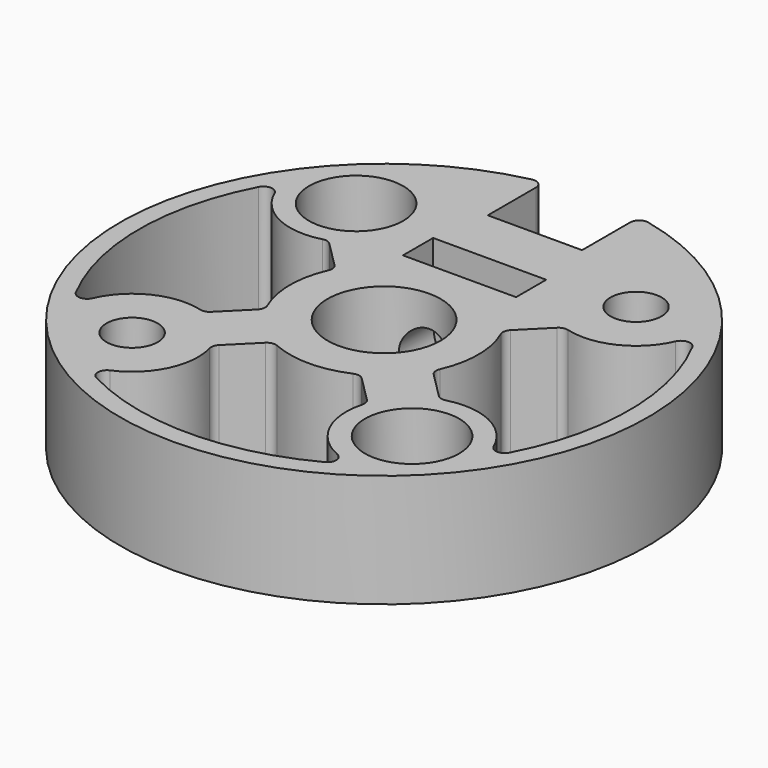
from build123d import *

# Parameters (mm, degrees)
F0_R            = 2.15265
F0_R_2          = 4.7625
F0_W            = 9.525
F0_H            = 3.175
F1_DEPTH        = 9.525
F2_R            = 2.15265
F3_REACH        = 44.1896136501
F6_R            = 3.96875
F7_DEPTH        = 6.35
F9_DEPTH        = 9.525
F9_COPIES_COUNT = 3
F9_COPIES_ANGLE = 180
F10_R           = 0.762
F12_R           = 3.96875
F13_DEPTH       = 6.35


# Not quite as in the source:
# - a feature of the source that left no trace in its solid (it failed there, or was rolled back) is left out
# - a pattern or mirror of a feature is missing from the dataset's text; its kind, count and spacing are read off the source's solid


with BuildPart() as f1:
    # F0 (on Top) → F1 (new body)
    with BuildSketch(Plane.XY):
        with BuildLine():
            Line((3.96875, 15.875), (-3.96875, 15.875))
            Line((-3.96875, 15.875), (-3.96875, 21.8677764859))
            ThreePointArc((-3.96875, 21.8677764859), (0, -22.225), (3.96875, 21.8677764859))
            Line((3.96875, 21.8677764859), (3.96875, 15.875))
        make_face()
        with Locations((-11.7865861589, -11.7865861589)):
            Circle(F0_R, mode=Mode.SUBTRACT)
        with Locations((11.7865861589, -11.7865861589)):
            Circle(F0_R, mode=Mode.SUBTRACT)
        with Locations((-11.7865861589, 11.7865861589)):
            Circle(F0_R, mode=Mode.SUBTRACT)
        Circle(F0_R_2, mode=Mode.SUBTRACT)
        with Locations((0, 9.525)):
            Rectangle(F0_W, F0_H, mode=Mode.SUBTRACT)
        with Locations((11.7865861589, 11.7865861589)):
            Circle(F0_R, mode=Mode.SUBTRACT)
    extrude(amount=F1_DEPTH)

    f3_end = f1.faces().sort_by_distance((-4.7625, 0, 4.7625))[0]
    # F2 (on face) → F3 (cut, up to a face of the model that its end follows)
    with BuildSketch(Plane(origin=(0, 15.875, 0), x_dir=(-1, 0, 0), z_dir=(0, 1, 0))):
        with Locations((0, 4.7625)):
            Circle(F2_R)
    f3_long = extrude(amount=-F3_REACH, mode=Mode.PRIVATE)
    add(split(f3_long, bisect_by=f3_end, keep=Keep.ALL, mode=Mode.PRIVATE).solids().sort_by_distance((0, 15.875, 4.7625))[0], mode=Mode.SUBTRACT)

    # F6 (on face) → F7 (cut, through all)
    with BuildSketch(Plane(origin=(0, 0, 0), x_dir=(1, 0, 0), z_dir=(0, 0, -1))):
        with Locations((11.7865861589, -11.7865861589)):
            Circle(F6_R)
        with Locations((-11.7865861589, 11.7865861589)):
            Circle(F6_R)
    extrude(amount=-F7_DEPTH, mode=Mode.SUBTRACT)

    # F8 (on face) → F9 (cut, through all)
    with BuildSketch(Plane(origin=(0, 0, 0), x_dir=(1, 0, 0), z_dir=(0, 0, -1))):
        with BuildLine():
            ThreePointArc((-17.3148424047, -11.229543123), (-14.7565267097, -7.0906978311), (-9.9206262673, -6.5530302219))
            Line((-9.9206262673, -6.5530302219), (-7.0379344931, -3.6703384477))
            ThreePointArc((-7.0379344931, -3.6703384477), (-7.9375, 0), (-7.0379344931, 3.6703384477))
            Line((-7.0379344931, 3.6703384477), (-9.9206262673, 6.5530302219))
            ThreePointArc((-9.9206262673, 6.5530302219), (-14.7565267097, 7.0906978311), (-17.3148424047, 11.229543123))
            ThreePointArc((-17.3148424047, 11.229543123), (-20.6375, 0), (-17.3148424047, -11.229543123))
        make_face()
    f9 = extrude(amount=-F9_DEPTH, mode=Mode.SUBTRACT)

    # F9_copies: F9 ×3 about axis
    f9_copies_axis = Axis((0, 0, 0), (0, 0, 1))
    for i in range(1, F9_COPIES_COUNT):
        add(f9.rotate(f9_copies_axis, i * F9_COPIES_ANGLE / (F9_COPIES_COUNT - 1)), mode=Mode.SUBTRACT)

    # F10
    f10_edges = [f1.edges().sort_by_distance(p)[0] for p in [
        (-17.314842, -11.229543, 4.7625),
        (-9.920626, -6.55303, 4.7625),
        (-7.037934, -3.670338, 4.7625),
        (-7.037934, 3.670338, 4.7625),
        (-9.920626, 6.55303, 4.7625),
        (-17.314842, 11.229543, 4.7625),
        (3.96875, 21.867776, 4.7625),
        (-3.96875, 21.867776, 4.7625),
        (11.229543, -17.314842, 4.7625),
        (-11.229543, -17.314842, 4.7625),
        (6.55303, -9.920626, 4.7625),
        (-6.55303, -9.920626, 4.7625),
        (3.670338, -7.037934, 4.7625),
        (-3.670338, -7.037934, 4.7625),
        (17.314842, 11.229543, 4.7625),
        (17.314842, -11.229543, 4.7625),
        (9.920626, 6.55303, 4.7625),
        (7.037934, 3.670338, 4.7625),
        (7.037934, -3.670338, 4.7625),
        (9.920626, -6.55303, 4.7625),
    ]]
    fillet(f10_edges, radius=F10_R)

    # F12 (on face) → F13 (cut, through all)
    with BuildSketch(Plane.XY.offset(9.525)):
        with Locations((11.7865861589, -11.7865861589)):
            Circle(F12_R)
        with Locations((-11.7865861589, 11.7865861589)):
            Circle(F12_R)
    extrude(amount=-F13_DEPTH, mode=Mode.SUBTRACT)


solid = f1.part
